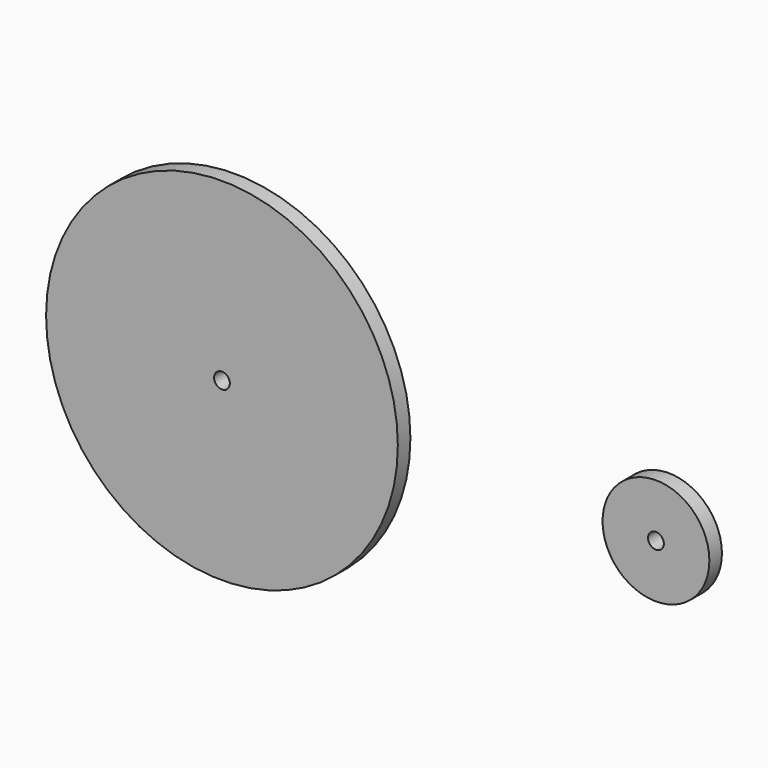
from build123d import *

# Parameters (mm, degrees)
F0_R     = 35.56
F0_R_2   = 1.59385
F1_DEPTH = 1.5875
F0_R_3   = 10.795


# Not quite as in the source:
# - a length typed as a fraction of an inch, garbled in the dataset ("3 / 203.2 mm" for 3/8 in), is restored


with BuildPart() as f1:
    # F0 (on Front) → F1 (new body, symmetric)
    with BuildSketch(Plane.XZ):
        with Locations((-53.3297125294, 0)):
            Circle(F0_R)
        with Locations((-53.3297125294, 0)):
            Circle(F0_R_2, mode=Mode.SUBTRACT)
    extrude(amount=F1_DEPTH, both=True)


with BuildPart() as f1b:
    # F0 (on Front) → F1, piece 2 (new body, symmetric)
    with BuildSketch(Plane.XZ):
        with Locations((34.4214282293, 0)):
            Circle(F0_R_3)
        with Locations((34.4214282293, 0)):
            Circle(F0_R_2, mode=Mode.SUBTRACT)
    extrude(amount=F1_DEPTH, both=True)


solid = Compound([f1.part, f1b.part])
